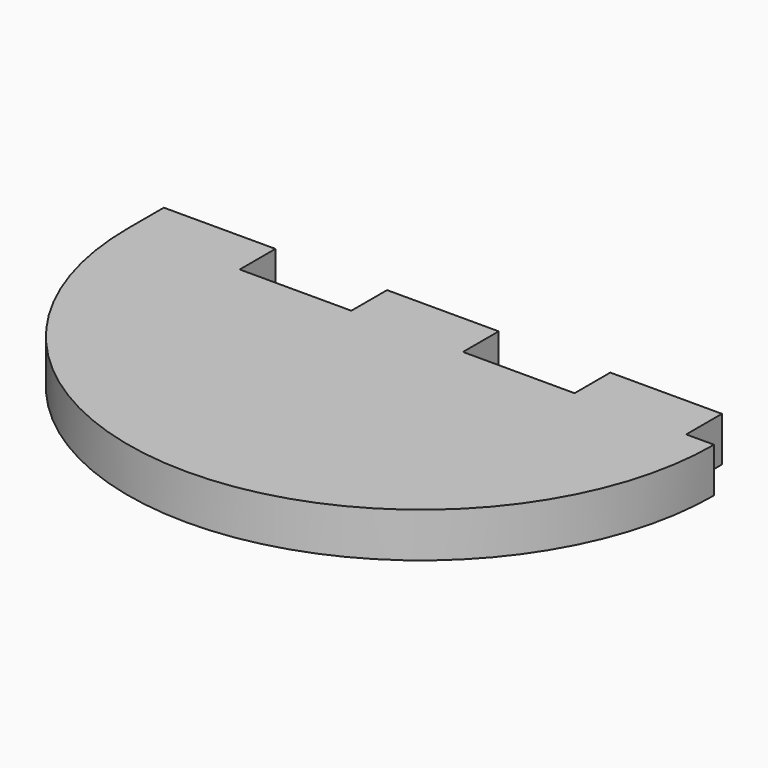
from build123d import *

# Parameters (mm, degrees)
F1_DEPTH = 1.6


# Not quite as in the source:
# - a feature names something its author has since deleted; it is built from what else it names


with BuildPart() as f1:
    # F0 (on Top) → F1 (new body, symmetric)
    with BuildSketch(Plane.XY):
        with BuildLine():
            Line((-21, 3.2), (-21, 0))
            ThreePointArc((-21, 0), (0, -21), (21, 0))
            Line((21, 0), (19, 0))
            Line((19, 0), (19, 3.2))
            Line((19, 3.2), (11, 3.2))
            Line((11, 3.2), (11, 0))
            Line((11, 0), (3, 0))
            Line((3, 0), (3, 3.2))
            Line((3, 3.2), (-5, 3.2))
            Line((-5, 3.2), (-5, 0))
            Line((-5, 0), (-13, 0))
            Line((-13, 0), (-13, 3.2))
            Line((-13, 3.2), (-21, 3.2))
        make_face()
    extrude(amount=F1_DEPTH, both=True)


solid = f1.part
